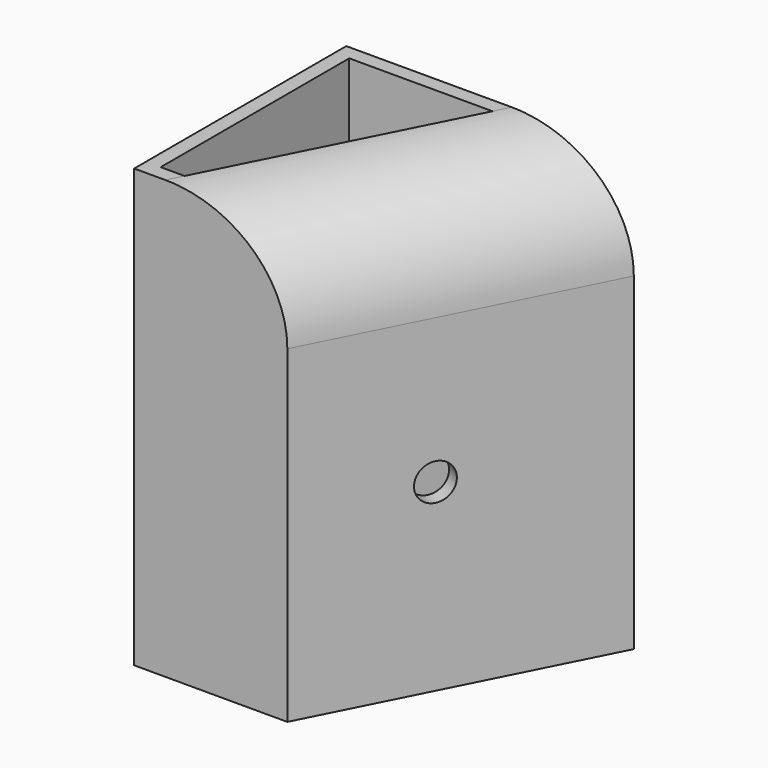
from build123d import *

# Parameters (mm, degrees)
F1_DEPTH = 75.438
F2_R     = 18.7791754174
F3_T     = -2.54
F5_D     = 6.35


# Not quite as in the source:
# - a shell that OpenCascade refuses in one call is made with other operations: the cavity is built on its own and cut out


with BuildPart() as f1:
    # F0 (on Top) → F1 (new body)
    with BuildSketch(Plane.XY):
        Polygon((0, 45.7287728786), (0, 0), (26.4172311872, 0), (49.5915971696, 45.7287728786), align=None)
    extrude(amount=F1_DEPTH)

    # F2
    f2_edges = [f1.edges().sort_by_distance(p)[0] for p in [
        (38.004414, 22.864386, 75.438),
    ]]
    fillet(f2_edges, radius=F2_R)

    # F3: a shell. OpenCascade refuses it in one call, so the cavity is built on its own and cut out:
    # the body offset inwards by the wall thickness, plus a prism from it out through each open face.
    f3_core = offset(f1.part, amount=F3_T, kind=Kind.INTERSECTION, mode=Mode.PRIVATE)
    f3_exits = [f3_core.faces().sort_by_distance(p)[0] for p in [
        (10.972623, 27.706391, 72.898),
    ]]
    add(f3_core, mode=Mode.SUBTRACT)
    extrude(f3_exits, amount=-F3_T, mode=Mode.SUBTRACT)

    # F5 (through all)
    with Locations(Plane(origin=(21.0190277096, -10.6519945775, 0), x_dir=(0.4520442786, 0.891995499, 0), z_dir=(0.891995499, -0.4520442786, 0))):
        with Locations((33.8537804782, 31.7050926387)):
            Hole(F5_D / 2)


solid = f1.part
